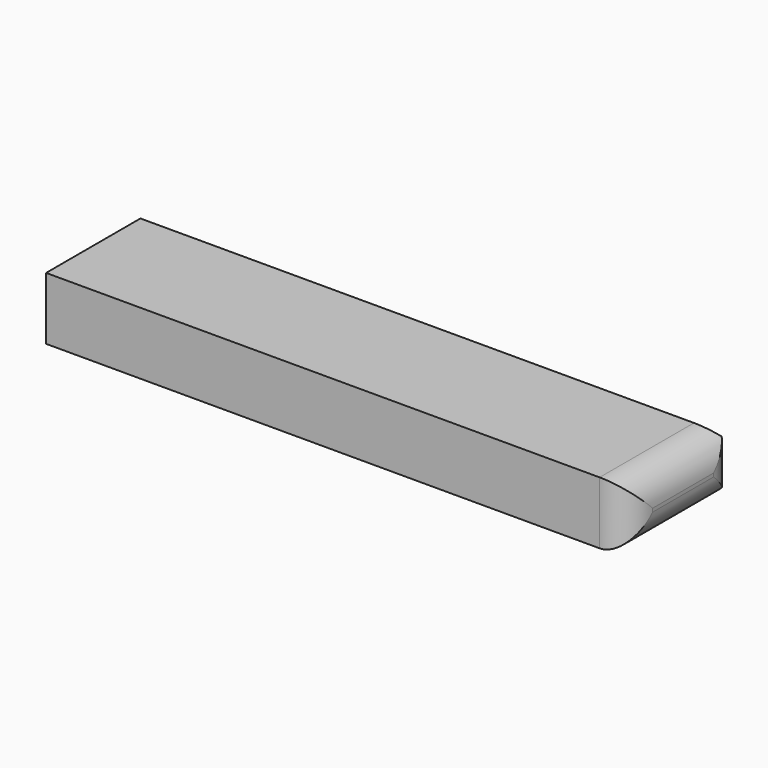
from build123d import *

# Parameters (mm, degrees)
F1_DEPTH    = 1.27
F2_W        = 50.2304956317
F2_H        = 5.3818384185
F3_DEPTH    = 12.7
F5_SIZE     = 2.54
F6_T1_DEPTH = 22.86
F6_T3_DEPTH = 10.6423506607
F6_T5_DEPTH = 18.0818384185


# Not quite as in the source:
# - a fillet or chamfer that OpenCascade refuses, or shapes differently, is made with other operations: its cross-section is extruded or revolved along the edge and cut away or added


with BuildPart() as f1:
    # F0 (on Front) → F1 (new body)
    with BuildSketch(Plane.XZ):
        with BuildLine():
            ThreePointArc((3.2290674407, 2.4202670825), (3.8285241608, 1.2755281407), (4.0354143885, 0))
            ThreePointArc((4.0354143885, 0), (3.8285241608, -1.2755281407), (3.2290674407, -2.4202670825))
            Line((3.2290674407, -2.4202670825), (3.2290674407, -2.6700689923))
            Line((3.2290674407, -2.6700689923), (53.7696667016, -2.6700689923))
            Line((53.7696667016, -2.6700689923), (53.7696667016, 2.4202670825))
            Line((53.7696667016, 2.4202670825), (3.2290674407, 2.4202670825))
        make_face()
    extrude(amount=F1_DEPTH)


with BuildPart() as f3:
    # F2 (on face) → F3 (new body)
    with BuildSketch(Plane.XZ.offset(1.27)):
        with Locations((-25.1152478158, 2.6909192093)):
            Rectangle(F2_W, F2_H)
    extrude(amount=F3_DEPTH)

    # F5
    f5_edges = [f3.edges().sort_by_distance(p)[0] for p in [
        (-25.115248, -1.27, 0),
        (0, -1.27, 2.690919),
        (-25.115248, -1.27, 5.381838),
        (-50.230496, -1.27, 2.690919),
    ]]
    chamfer(f5_edges, length=F5_SIZE)

    # F6: fillet of radius 2.54 on 4 edges, made by hand

    # F6_s2 → F6_t1 (cut)
    with BuildSketch(Plane.XZ.offset(-2.54)):
        with BuildLine():
            ThreePointArc((-2.54, 0), (-0.7439487758, 0.7439487758), (0, 2.54))
            Line((0, 2.54), (0, 0))
            Line((0, 0), (-2.54, 0))
        make_face()
        with BuildLine():
            ThreePointArc((0, 2.8418384185), (-0.7439487758, 4.6378896428), (-2.54, 5.3818384185))
            Line((-2.54, 5.3818384185), (0, 5.3818384185))
            Line((0, 5.3818384185), (0, 2.8418384185))
        make_face()
    extrude(amount=F6_T1_DEPTH, mode=Mode.SUBTRACT)

    # F6_s4 → F6_t3 (cut)
    with BuildSketch(Plane.XY.offset(-2.6302561211)):
        with BuildLine():
            ThreePointArc((0, -4.8621024484), (-0.1933459874, -3.8900865302), (-0.7439487758, -3.0660512242))
            Line((-0.7439487758, -3.0660512242), (0, -3.81))
            Line((0, -3.81), (0, -4.8621024484))
        make_face()
    extrude(amount=F6_T3_DEPTH, mode=Mode.SUBTRACT)

    # F6_s6 → F6_t5 (cut)
    with BuildSketch(Plane.XY.offset(-6.35)):
        with BuildLine():
            ThreePointArc((-2.54, -13.97), (-0.7439487758, -13.2260512242), (0, -11.43))
            Line((0, -11.43), (0, -13.97))
            Line((0, -13.97), (-2.54, -13.97))
        make_face()
    extrude(amount=F6_T5_DEPTH, mode=Mode.SUBTRACT)


solid = f3.part
